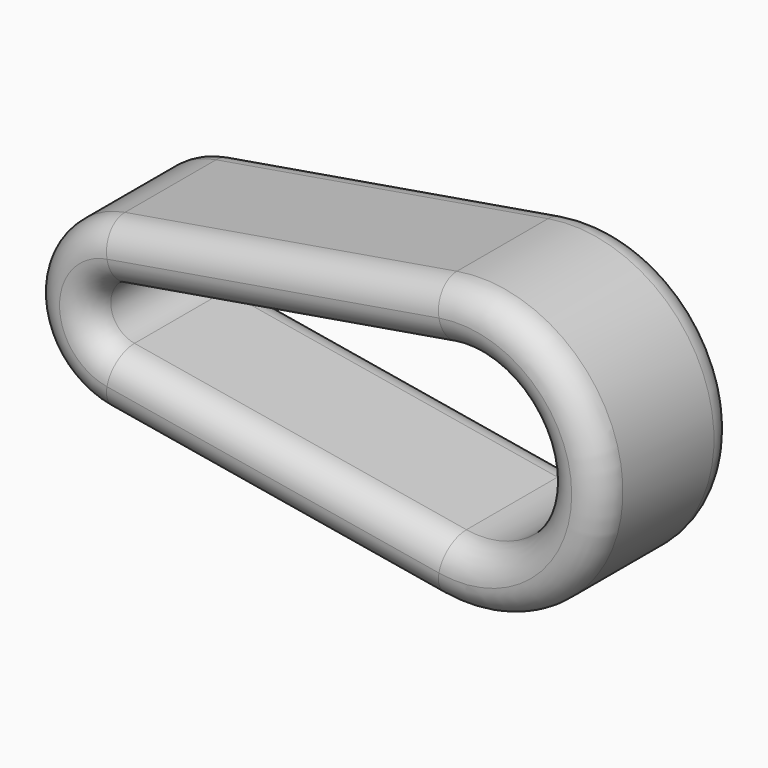
from build123d import *

# Parameters (mm, degrees)
F1_DEPTH      = 15
F1_DEPTH_BACK = 15
F2_R          = 4.99999


# Not quite as in the source:
# - a fillet or chamfer is up to 0.001 mm smaller than in the source, because OpenCascade refuses the exact size


with BuildPart() as f1:
    # F0 (on Front) → F1 (new body, two sides)
    with BuildSketch(Plane.XZ) as f1_sk:
        with BuildLine():
            Line((-2.5, -14.7901994577), (55.8333333333, -24.6503324296))
            ThreePointArc((55.8333333333, -24.6503324296), (85, 0), (55.8333333333, 24.6503324296))
            Line((55.8333333333, 24.6503324296), (-2.5, 14.7901994577))
            ThreePointArc((-2.5, 14.7901994577), (-15, 0), (-2.5, -14.7901994577))
        make_face()
        with BuildLine():
            ThreePointArc((-0.8333333333, -4.9300664859), (-5, 0), (-0.8333333333, 4.9300664859))
            Line((-0.8333333333, 4.9300664859), (57.5, 14.7901994577))
            ThreePointArc((57.5, 14.7901994577), (75, 0), (57.5, -14.7901994577))
            Line((57.5, -14.7901994577), (-0.8333333333, -4.9300664859))
        make_face(mode=Mode.SUBTRACT)
    extrude(amount=F1_DEPTH)
    extrude(f1_sk.sketch, amount=-F1_DEPTH_BACK)

    # F2 (radius 5 in the source; OpenCascade refuses exactly that, so slightly less here)
    f2_edges = [f1.edges().sort_by_distance(p)[0] for p in [
        (28.333333, -15, 9.860133),
        (26.666667, -15, 19.720266),
        (26.666667, 15, 19.720266),
        (28.333333, 15, 9.860133),
    ]]
    fillet(f2_edges, radius=F2_R)


solid = f1.part
